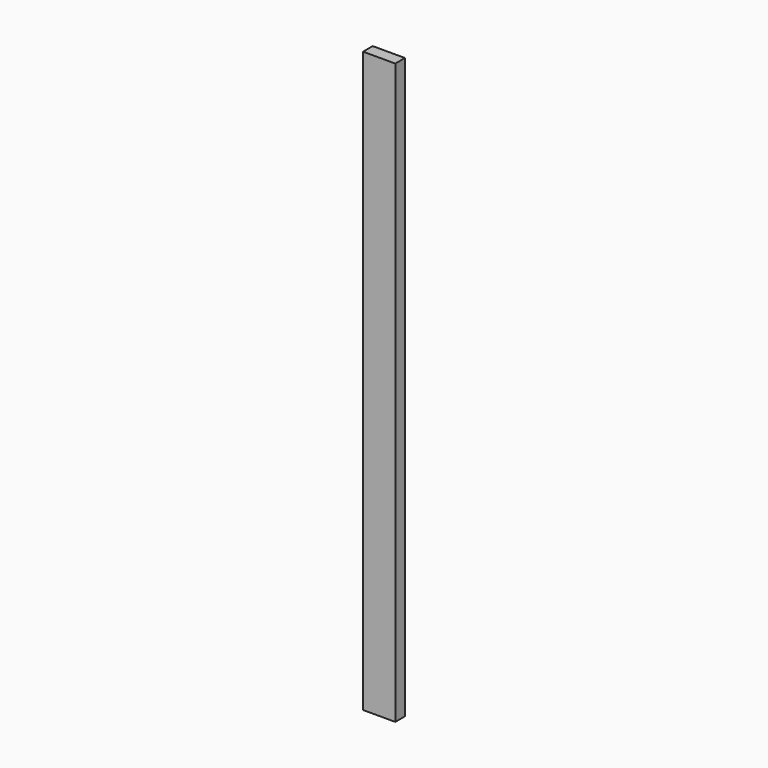
from build123d import *

# Parameters (mm, degrees)
F0_W     = 50.8
F0_H     = 914.4
F1_DEPTH = 19.05


# Not quite as in the source:
# - a length typed as a fraction of an inch, garbled in the dataset ("3 / 203.2 mm" for 3/8 in), is restored


with BuildPart() as f1:
    # F0 (on Front) → F1 (new body)
    with BuildSketch(Plane.XZ):
        with Locations((-29.3033250332, 33.3588020876)):
            Rectangle(F0_W, F0_H)
    extrude(amount=F1_DEPTH)


solid = f1.part
